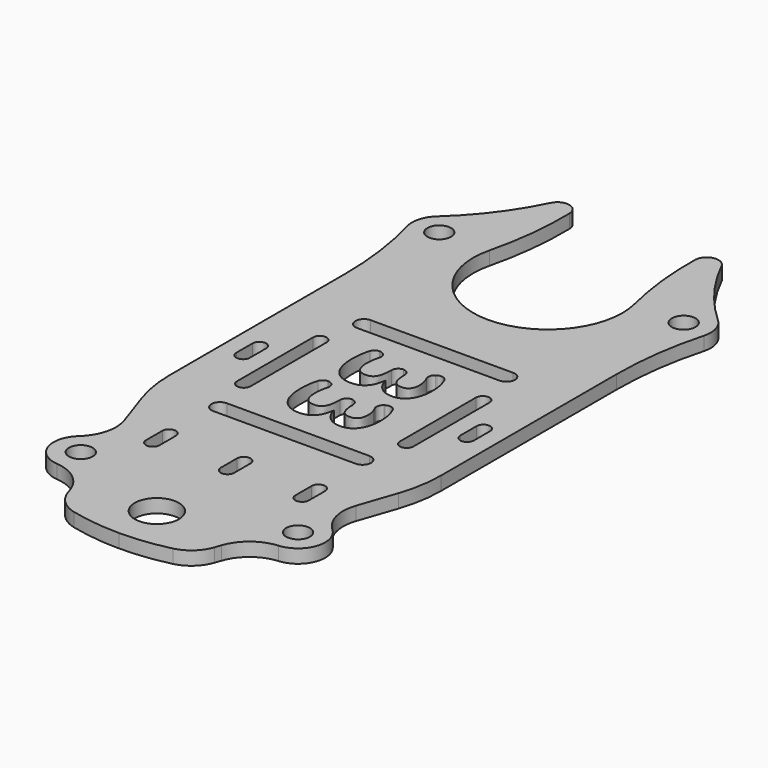
from build123d import *

# Parameters (mm, degrees)
F0_R        = 1.75
F0_R_2      = 3.25
F1_DEPTH    = 2
F2_T1_DEPTH = 2
F4_DEPTH    = 25


# Not quite as in the source:
# - a fillet or chamfer that OpenCascade refuses, or shapes differently, is made with other operations: its cross-section is extruded or revolved along the edge and cut away or added


with BuildPart() as f1:
    # F0 (on Top) → F1 (new body)
    with BuildSketch(Plane.XY):
        with BuildLine():
            ThreePointArc((-12.5713700234, 50.2695594093), (-16.118909248, 44.4802706126), (-20.6903729233, 39.460049583))
            ThreePointArc((-20.6903729233, 39.460049583), (-21.8414318775, 37.6150789796), (-21.8571428571, 35.4405430733))
            ThreePointArc((-21.8571428571, 35.4405430733), (-20.4663771338, 28.6163953155), (-20, 21.6676030258))
            Line((-20, 21.6676030258), (-20, -10.6856030045))
            ThreePointArc((-20, -10.6856030045), (-19.7308995433, -13.9554047127), (-18.9308396789, -17.1372159077))
            Line((-18.9308396789, -17.1372159077), (-17.0470641697, -22.6647409918))
            ThreePointArc((-17.0470641697, -22.6647409918), (-16.9162578432, -26.0979642803), (-18.6905264293, -29.0400899451))
            ThreePointArc((-18.6905264293, -29.0400899451), (-19.7861679358, -33.2903225806), (-16.3230484377, -35.9869336221))
            ThreePointArc((-16.3230484377, -35.9869336221), (-13.1213600073, -37.2332576723), (-11.1283691906, -40.0318501842))
            Line((-11.1283691906, -40.0318501842), (-10.837240035, -40.8861046865))
            ThreePointArc((-10.837240035, -40.8861046865), (-9.4747581102, -42.9666501557), (-7.2784782144, -44.1334325108))
            ThreePointArc((-7.2784782144, -44.1334325108), (-3.6649414842, -44.7825957956), (0, -45))
            ThreePointArc((0, -45), (3.6649414842, -44.7825957956), (7.2784782144, -44.1334325108))
            ThreePointArc((7.2784782144, -44.1334325108), (9.4747581102, -42.9666501557), (10.837240035, -40.8861046865))
            Line((10.837240035, -40.8861046865), (11.1283691906, -40.0318501842))
            ThreePointArc((11.1283691906, -40.0318501842), (13.1213600073, -37.2332576723), (16.3230484377, -35.9869336221))
            ThreePointArc((16.3230484377, -35.9869336221), (19.7861679358, -33.2903225806), (18.6905264293, -29.0400899451))
            ThreePointArc((18.6905264293, -29.0400899451), (16.9162578432, -26.0979642803), (17.0470641697, -22.6647409918))
            Line((17.0470641697, -22.6647409918), (18.9308396789, -17.1372159077))
            ThreePointArc((18.9308396789, -17.1372159077), (19.7308995433, -13.9554047127), (20, -10.6856030045))
            Line((20, -10.6856030045), (20, 21.6676030258))
            ThreePointArc((20, 21.6676030258), (20.4663771338, 28.6163953155), (21.8571428571, 35.4405430733))
            ThreePointArc((21.8571428571, 35.4405430733), (21.8414318775, 37.6150789796), (20.6903729233, 39.460049583))
            ThreePointArc((20.6903729233, 39.460049583), (16.118909248, 44.4802706126), (12.5713700234, 50.2695594093))
            ThreePointArc((12.5713700234, 50.2695594093), (10.6215560146, 51.2086657952), (9.25, 49.5345900586))
            ThreePointArc((9.25, 49.5345900586), (9.5452241746, 43.0321205381), (10.6826647736, 36.6231037599))
            ThreePointArc((10.6826647736, 36.6231037599), (8.6560424375, 27.2122957253), (0, 23))
            ThreePointArc((0, 23), (-8.6560424375, 27.2122957253), (-10.6826647736, 36.6231037599))
            ThreePointArc((-10.6826647736, 36.6231037599), (-9.5452241746, 43.0321205381), (-9.25, 49.5345900586))
            ThreePointArc((-9.25, 49.5345900586), (-10.6215560146, 51.2086657952), (-12.5713700234, 50.2695594093))
        make_face()
        with Locations((-16, -32)):
            Circle(F0_R, mode=Mode.SUBTRACT)
        with BuildLine():
            Line((-17.5, -1.5), (-17.5, 1.5))
            ThreePointArc((-17.5, 1.5), (-16.5, 2.5), (-15.5, 1.5))
            Line((-15.5, 1.5), (-15.5, -1.5))
            ThreePointArc((-15.5, -1.5), (-16.5, -2.5), (-17.5, -1.5))
        make_face(mode=Mode.SUBTRACT)
        with BuildLine():
            Line((-13, -7), (-13, 7))
            ThreePointArc((-13, 7), (-12, 8), (-11, 7))
            Line((-11, 7), (-11, -7))
            ThreePointArc((-11, -7), (-12, -8), (-13, -7))
        make_face(mode=Mode.SUBTRACT)
        with BuildLine():
            add(Edge.make_bspline(
                [(5.3190104167, -7.2317708333), (4.5703125, -8.3020833333), (3.2369791667, -8.3020833333)],
                knots=[0, 0, 0, 1, 1, 1], degree=2))
            add(Edge.make_bspline(
                [(3.2369791667, -8.3020833333), (2.1223958333, -8.3020833333), (1.3411458333, -7.6263020833)],
                knots=[0, 0, 0, 1, 1, 1], degree=2))
            add(Edge.make_bspline(
                [(1.3411458333, -7.6263020833), (0.5598958333, -6.9505208333), (0.265625, -5.7291666667)],
                knots=[0, 0, 0, 1, 1, 1], degree=2))
            Line((0.265625, -5.7291666667), (0.21875, -5.7291666667))
            add(Edge.make_bspline(
                [(0.21875, -5.7291666667), (0.0390625, -7.171875), (-0.6575520833, -7.9114583333)],
                knots=[0, 0, 0, 1, 1, 1], degree=2))
            add(Edge.make_bspline(
                [(-0.6575520833, -7.9114583333), (-1.3541666667, -8.6510416667), (-2.5338541667, -8.6510416667)],
                knots=[0, 0, 0, 1, 1, 1], degree=2))
            add(Edge.make_bspline(
                [(-2.5338541667, -8.6510416667), (-4.25, -8.6510416667), (-5.20703125, -7.40625)],
                knots=[0, 0, 0, 1, 1, 1], degree=2))
            add(Edge.make_bspline(
                [(-5.20703125, -7.40625), (-6.1640625, -6.1614583333), (-6.1640625, -3.8515625)],
                knots=[0, 0, 0, 1, 1, 1], degree=2))
            add(Edge.make_bspline(
                [(-6.1640625, -3.8515625), (-6.1640625, -1.9140625), (-5.5208333333, -0.4166666667)],
                knots=[0, 0, 0, 1, 1, 1], degree=2))
            Line((-5.5208333333, -0.4166666667), (-3.3802083333, -0.4166666667))
            add(Edge.make_bspline(
                [(-3.3802083333, -0.4166666667), (-3.7291666667, -1.1067708333), (-3.94921875, -1.9375)],
                knots=[0, 0, 0, 1, 1, 1], degree=2))
            add(Edge.make_bspline(
                [(-3.94921875, -1.9375), (-4.1692708333, -2.7682291667), (-4.1692708333, -3.5807291667)],
                knots=[0, 0, 0, 1, 1, 1], degree=2))
            add(Edge.make_bspline(
                [(-4.1692708333, -3.5807291667), (-4.1692708333, -4.828125), (-3.74609375, -5.421875)],
                knots=[0, 0, 0, 1, 1, 1], degree=2))
            add(Edge.make_bspline(
                [(-3.74609375, -5.421875), (-3.3229166667, -6.015625), (-2.3854166667, -6.015625)],
                knots=[0, 0, 0, 1, 1, 1], degree=2))
            add(Edge.make_bspline(
                [(-2.3854166667, -6.015625), (-1.5494791667, -6.015625), (-1.19921875, -5.33203125)],
                knots=[0, 0, 0, 1, 1, 1], degree=2))
            add(Edge.make_bspline(
                [(-1.19921875, -5.33203125), (-0.8489583333, -4.6484375), (-0.8489583333, -3.1510416667)],
                knots=[0, 0, 0, 1, 1, 1], degree=2))
            Line((-0.8489583333, -3.1510416667), (-0.8489583333, -2.2473958333))
            Line((-0.8489583333, -2.2473958333), (1.0807291667, -2.2473958333))
            Line((1.0807291667, -2.2473958333), (1.0807291667, -3.1666666667))
            add(Edge.make_bspline(
                [(1.0807291667, -3.1666666667), (1.0807291667, -4.5494791667), (1.4427083333, -5.1888020833)],
                knots=[0, 0, 0, 1, 1, 1], degree=2))
            add(Edge.make_bspline(
                [(1.4427083333, -5.1888020833), (1.8046875, -5.828125), (2.6822916667, -5.828125)],
                knots=[0, 0, 0, 1, 1, 1], degree=2))
            add(Edge.make_bspline(
                [(2.6822916667, -5.828125), (4.0338541667, -5.828125), (4.0338541667, -4.1354166667)],
                knots=[0, 0, 0, 1, 1, 1], degree=2))
            add(Edge.make_bspline(
                [(4.0338541667, -4.1354166667), (4.0338541667, -3.5494791667), (3.8385416667, -2.9427083333)],
                knots=[0, 0, 0, 1, 1, 1], degree=2))
            add(Edge.make_bspline(
                [(3.8385416667, -2.9427083333), (3.6432291667, -2.3359375), (3.1640625, -1.5963541667)],
                knots=[0, 0, 0, 1, 1, 1], degree=2))
            Line((3.1640625, -1.5963541667), (4.8958333333, -0.4322916667))
            add(Edge.make_bspline(
                [(4.8958333333, -0.4322916667), (6.0677083333, -2.0598958333), (6.0677083333, -4.3151041667)],
                knots=[0, 0, 0, 1, 1, 1], degree=2))
            add(Edge.make_bspline(
                [(6.0677083333, -4.3151041667), (6.0677083333, -6.1614583333), (5.3190104167, -7.2317708333)],
                knots=[0, 0, 0, 1, 1, 1], degree=2))
        make_face(mode=Mode.SUBTRACT)
        with Locations((0, -38)):
            Circle(F0_R_2, mode=Mode.SUBTRACT)
        with Locations((16, -32)):
            Circle(F0_R, mode=Mode.SUBTRACT)
        with BuildLine():
            Line((10.5, -14.5), (-10.5, -14.5))
            ThreePointArc((-10.5, -14.5), (-11.75, -13.25), (-10.5, -12))
            Line((-10.5, -12), (10.5, -12))
            ThreePointArc((10.5, -12), (11.75, -13.25), (10.5, -14.5))
        make_face(mode=Mode.SUBTRACT)
        with BuildLine():
            Line((11, -7), (11, 7))
            ThreePointArc((11, 7), (12, 8), (13, 7))
            Line((13, 7), (13, -7))
            ThreePointArc((13, -7), (12, -8), (11, -7))
        make_face(mode=Mode.SUBTRACT)
        with BuildLine():
            Line((15.5, -1.5), (15.5, 1.5))
            ThreePointArc((15.5, 1.5), (16.5, 2.5), (17.5, 1.5))
            Line((17.5, 1.5), (17.5, -1.5))
            ThreePointArc((17.5, -1.5), (16.5, -2.5), (15.5, -1.5))
        make_face(mode=Mode.SUBTRACT)
        with BuildLine():
            add(Edge.make_bspline(
                [(5.3190104167, 2.28125), (4.5703125, 1.2109375), (3.2369791667, 1.2109375)],
                knots=[0, 0, 0, 1, 1, 1], degree=2))
            add(Edge.make_bspline(
                [(3.2369791667, 1.2109375), (2.1223958333, 1.2109375), (1.3411458333, 1.88671875)],
                knots=[0, 0, 0, 1, 1, 1], degree=2))
            add(Edge.make_bspline(
                [(1.3411458333, 1.88671875), (0.5598958333, 2.5625), (0.265625, 3.7838541667)],
                knots=[0, 0, 0, 1, 1, 1], degree=2))
            Line((0.265625, 3.7838541667), (0.21875, 3.7838541667))
            add(Edge.make_bspline(
                [(0.21875, 3.7838541667), (0.0390625, 2.3411458333), (-0.6575520833, 1.6015625)],
                knots=[0, 0, 0, 1, 1, 1], degree=2))
            add(Edge.make_bspline(
                [(-0.6575520833, 1.6015625), (-1.3541666667, 0.8619791667), (-2.5338541667, 0.8619791667)],
                knots=[0, 0, 0, 1, 1, 1], degree=2))
            add(Edge.make_bspline(
                [(-2.5338541667, 0.8619791667), (-4.25, 0.8619791667), (-5.20703125, 2.1067708333)],
                knots=[0, 0, 0, 1, 1, 1], degree=2))
            add(Edge.make_bspline(
                [(-5.20703125, 2.1067708333), (-6.1640625, 3.3515625), (-6.1640625, 5.6614583333)],
                knots=[0, 0, 0, 1, 1, 1], degree=2))
            add(Edge.make_bspline(
                [(-6.1640625, 5.6614583333), (-6.1640625, 7.5989583333), (-5.5208333333, 9.0963541667)],
                knots=[0, 0, 0, 1, 1, 1], degree=2))
            Line((-5.5208333333, 9.0963541667), (-3.3802083333, 9.0963541667))
            add(Edge.make_bspline(
                [(-3.3802083333, 9.0963541667), (-3.7291666667, 8.40625), (-3.94921875, 7.5755208333)],
                knots=[0, 0, 0, 1, 1, 1], degree=2))
            add(Edge.make_bspline(
                [(-3.94921875, 7.5755208333), (-4.1692708333, 6.7447916667), (-4.1692708333, 5.9322916667)],
                knots=[0, 0, 0, 1, 1, 1], degree=2))
            add(Edge.make_bspline(
                [(-4.1692708333, 5.9322916667), (-4.1692708333, 4.6848958333), (-3.74609375, 4.0911458333)],
                knots=[0, 0, 0, 1, 1, 1], degree=2))
            add(Edge.make_bspline(
                [(-3.74609375, 4.0911458333), (-3.3229166667, 3.4973958333), (-2.3854166667, 3.4973958333)],
                knots=[0, 0, 0, 1, 1, 1], degree=2))
            add(Edge.make_bspline(
                [(-2.3854166667, 3.4973958333), (-1.5494791667, 3.4973958333), (-1.19921875, 4.1809895833)],
                knots=[0, 0, 0, 1, 1, 1], degree=2))
            add(Edge.make_bspline(
                [(-1.19921875, 4.1809895833), (-0.8489583333, 4.8645833333), (-0.8489583333, 6.3619791667)],
                knots=[0, 0, 0, 1, 1, 1], degree=2))
            Line((-0.8489583333, 6.3619791667), (-0.8489583333, 7.265625))
            Line((-0.8489583333, 7.265625), (1.0807291667, 7.265625))
            Line((1.0807291667, 7.265625), (1.0807291667, 6.3463541667))
            add(Edge.make_bspline(
                [(1.0807291667, 6.3463541667), (1.0807291667, 4.9635416667), (1.4427083333, 4.32421875)],
                knots=[0, 0, 0, 1, 1, 1], degree=2))
            add(Edge.make_bspline(
                [(1.4427083333, 4.32421875), (1.8046875, 3.6848958333), (2.6822916667, 3.6848958333)],
                knots=[0, 0, 0, 1, 1, 1], degree=2))
            add(Edge.make_bspline(
                [(2.6822916667, 3.6848958333), (4.0338541667, 3.6848958333), (4.0338541667, 5.3776041667)],
                knots=[0, 0, 0, 1, 1, 1], degree=2))
            add(Edge.make_bspline(
                [(4.0338541667, 5.3776041667), (4.0338541667, 5.9635416667), (3.8385416667, 6.5703125)],
                knots=[0, 0, 0, 1, 1, 1], degree=2))
            add(Edge.make_bspline(
                [(3.8385416667, 6.5703125), (3.6432291667, 7.1770833333), (3.1640625, 7.9166666667)],
                knots=[0, 0, 0, 1, 1, 1], degree=2))
            Line((3.1640625, 7.9166666667), (4.8958333333, 9.0807291667))
            add(Edge.make_bspline(
                [(4.8958333333, 9.0807291667), (6.0677083333, 7.453125), (6.0677083333, 5.1979166667)],
                knots=[0, 0, 0, 1, 1, 1], degree=2))
            add(Edge.make_bspline(
                [(6.0677083333, 5.1979166667), (6.0677083333, 3.3515625), (5.3190104167, 2.28125)],
                knots=[0, 0, 0, 1, 1, 1], degree=2))
        make_face(mode=Mode.SUBTRACT)
        with Locations((-18, 36.5)):
            Circle(F0_R, mode=Mode.SUBTRACT)
        with BuildLine():
            Line((10.5, 12), (-10.5, 12))
            ThreePointArc((-10.5, 12), (-11.75, 13.25), (-10.5, 14.5))
            Line((-10.5, 14.5), (10.5, 14.5))
            ThreePointArc((10.5, 14.5), (11.75, 13.25), (10.5, 12))
        make_face(mode=Mode.SUBTRACT)
        with Locations((18, 36.5)):
            Circle(F0_R, mode=Mode.SUBTRACT)
    extrude(amount=F1_DEPTH)

    # F2: fillet of radius 1 on 12 edges, made by hand

    # F2_s2 → F2_t1 (join)
    with BuildSketch(Plane.XY):
        with BuildLine():
            ThreePointArc((5.4823401509, 8.0731777614), (4.843595419, 8.6204570948), (4.0129893365, 8.4877806577))
            Line((4.0129893365, 8.4877806577), (3.9571236712, 8.5708917705))
            ThreePointArc((3.9571236712, 8.5708917705), (4.3986572425, 8.8672000385), (4.839967668, 9.1638402795))
            Line((4.839967668, 9.1638402795), (4.9771020437, 9.1392426381))
            ThreePointArc((4.9771020437, 9.1392426381), (5.3001177746, 8.6415597398), (5.573409567, 8.1148285845))
            Line((5.573409567, 8.1148285845), (5.4823401509, 8.0731777614))
        make_face()
        with BuildLine():
            ThreePointArc((3.9353958823, 8.4356238546), (3.5267558643, 7.8636788331), (3.5947276057, 7.1640449185))
            Line((3.5947276057, 7.1640449185), (3.5047965874, 7.119995944))
            ThreePointArc((3.5047965874, 7.119995944), (3.3039302948, 7.4968765259), (3.0800202169, 7.8622167368))
            Line((3.0800202169, 7.8622167368), (3.1081983093, 7.9997755857))
            ThreePointArc((3.1081983093, 7.9997755857), (3.4939765733, 8.2590881932), (3.8795316916, 8.5187327736))
            Line((3.8795316916, 8.5187327736), (3.9353958823, 8.4356238546))
        make_face()
        with BuildLine():
            ThreePointArc((1.0813955663, 6.2718756487), (0.7855723775, 6.9752785605), (0.0800558835, 7.266025))
            Line((0.0800558835, 7.266025), (0.0800558835, 7.3661615685))
            ThreePointArc((0.0800558835, 7.3661615685), (0.5803925251, 7.3657615685), (1.0807291667, 7.3657615685))
            Line((1.0807291667, 7.3657615685), (1.1808657352, 7.265625))
            ThreePointArc((1.1808657352, 7.265625), (1.1808657352, 6.3463541667), (1.1815295346, 6.2725972821))
            Line((1.1815295346, 6.2725972821), (1.0813955663, 6.2718756487))
        make_face()
        with BuildLine():
            ThreePointArc((0.1516589864, 7.266025), (-0.5538546526, 6.9752813949), (-0.8496806385, 6.2718836946))
            Line((-0.8496806385, 6.2718836946), (-0.9498146009, 6.2726061326))
            ThreePointArc((-0.9498146009, 6.2726061326), (-0.9490949019, 6.3619791667), (-0.9490949019, 7.265625))
            Line((-0.9490949019, 7.265625), (-0.8489583333, 7.3657615685))
            ThreePointArc((-0.8489583333, 7.3657615685), (-0.3486496735, 7.3657615685), (0.1516589864, 7.3661615685))
            Line((0.1516589864, 7.3661615685), (0.1516589864, 7.266025))
        make_face()
        with BuildLine():
            ThreePointArc((-3.8823882856, 7.8130958508), (-4.0409586866, 8.6953409018), (-4.8424375028, 9.0967541667))
            Line((-4.8424375028, 9.0967541667), (-4.8424375028, 9.1968381664))
            ThreePointArc((-4.8424375028, 9.1968381664), (-4.1113229181, 9.1964381664), (-3.3802083333, 9.1964381664))
            Line((-3.3802083333, 9.1964381664), (-3.2908936182, 9.0511912541))
            ThreePointArc((-3.2908936182, 9.0511912541), (-3.5673911757, 8.4298441391), (-3.7863833638, 7.784814019))
            Line((-3.7863833638, 7.784814019), (-3.8823882856, 7.8130958508))
        make_face()
        with BuildLine():
            ThreePointArc((-4.8235215119, 9.0967541667), (-5.4178362512, 8.9015689774), (-5.7807035945, 8.3920254967))
            Line((-5.7807035945, 8.3920254967), (-5.8764218027, 8.4217926297))
            ThreePointArc((-5.8764218027, 8.4217926297), (-5.7538395512, 8.7821164437), (-5.6129352586, 9.1359179502))
            Line((-5.6129352586, 9.1359179502), (-5.5208333333, 9.1965941667))
            ThreePointArc((-5.5208333333, 9.1965941667), (-5.1721774226, 9.1965941667), (-4.8235215119, 9.1969941667))
            Line((-4.8235215119, 9.1969941667), (-4.8235215119, 9.0967541667))
        make_face()
        with BuildLine():
            ThreePointArc((-3.8823882856, -1.6999249825), (-4.0409586866, -0.8176799315), (-4.8424375028, -0.4162666667))
            Line((-4.8424375028, -0.4162666667), (-4.8424375028, -0.3161826669))
            ThreePointArc((-4.8424375028, -0.3161826669), (-4.1113229181, -0.3165826669), (-3.3802083333, -0.3165826669))
            Line((-3.3802083333, -0.3165826669), (-3.2908936182, -0.4618295792))
            ThreePointArc((-3.2908936182, -0.4618295792), (-3.5673911757, -1.0831766942), (-3.7863833638, -1.7282068143))
            Line((-3.7863833638, -1.7282068143), (-3.8823882856, -1.6999249825))
        make_face()
        with BuildLine():
            ThreePointArc((-4.8235215119, -0.4162666667), (-5.4178362512, -0.611451856), (-5.7807035945, -1.1209953366))
            Line((-5.7807035945, -1.1209953366), (-5.8764218027, -1.0912282036))
            ThreePointArc((-5.8764218027, -1.0912282036), (-5.7538395512, -0.7309043896), (-5.6129352586, -0.3771028831))
            Line((-5.6129352586, -0.3771028831), (-5.5208333333, -0.3164266667))
            ThreePointArc((-5.5208333333, -0.3164266667), (-5.1721774226, -0.3164266667), (-4.8235215119, -0.3160266667))
            Line((-4.8235215119, -0.3160266667), (-4.8235215119, -0.4162666667))
        make_face()
        with BuildLine():
            ThreePointArc((0.1516589864, -2.2469958333), (-0.5538546526, -2.5377394384), (-0.8496806385, -3.2411371388))
            Line((-0.8496806385, -3.2411371388), (-0.9498146009, -3.2404147008))
            ThreePointArc((-0.9498146009, -3.2404147008), (-0.9490949019, -3.1510416667), (-0.9490949019, -2.2473958333))
            Line((-0.9490949019, -2.2473958333), (-0.8489583333, -2.1472592648))
            ThreePointArc((-0.8489583333, -2.1472592648), (-0.3486496735, -2.1472592648), (0.1516589864, -2.1468592648))
            Line((0.1516589864, -2.1468592648), (0.1516589864, -2.2469958333))
        make_face()
        with BuildLine():
            ThreePointArc((1.0813955663, -3.2411451846), (0.7855723775, -2.5377422728), (0.0800558835, -2.2469958333))
            Line((0.0800558835, -2.2469958333), (0.0800558835, -2.1468592648))
            ThreePointArc((0.0800558835, -2.1468592648), (0.5803925251, -2.1472592648), (1.0807291667, -2.1472592648))
            Line((1.0807291667, -2.1472592648), (1.1808657352, -2.2473958333))
            ThreePointArc((1.1808657352, -2.2473958333), (1.1808657352, -3.1666666667), (1.1815295346, -3.2404235512))
            Line((1.1815295346, -3.2404235512), (1.0813955663, -3.2411451846))
        make_face()
        with BuildLine():
            ThreePointArc((3.9353958823, -1.0773969787), (3.5267558643, -1.6493420003), (3.5947276057, -2.3489759148))
            Line((3.5947276057, -2.3489759148), (3.5047965874, -2.3930248894))
            ThreePointArc((3.5047965874, -2.3930248894), (3.3039302948, -2.0161443075), (3.0800202169, -1.6508040966))
            Line((3.0800202169, -1.6508040966), (3.1081983093, -1.5132452476))
            ThreePointArc((3.1081983093, -1.5132452476), (3.4939765733, -1.2539326401), (3.8795316916, -0.9942880597))
            Line((3.8795316916, -0.9942880597), (3.9353958823, -1.0773969787))
        make_face()
        with BuildLine():
            ThreePointArc((4.0129893365, -1.0252401757), (4.843595419, -0.8925637385), (5.4823401509, -1.439843072))
            Line((5.4823401509, -1.439843072), (5.573409567, -1.3981922488))
            ThreePointArc((5.573409567, -1.3981922488), (5.3001177746, -0.8714610935), (4.9771020437, -0.3737781952))
            Line((4.9771020437, -0.3737781952), (4.839967668, -0.3491805539))
            ThreePointArc((4.839967668, -0.3491805539), (4.3986572425, -0.6458207948), (3.9571236712, -0.9421290629))
            Line((3.9571236712, -0.9421290629), (4.0129893365, -1.0252401757))
        make_face()
    extrude(amount=F2_T1_DEPTH)

    # F3 (on face) → F4 (cut)
    with BuildSketch(Plane.XY.offset(2)):
        with BuildLine():
            ThreePointArc((12, -22), (11, -21), (10, -22))
            Line((10, -22), (10, -25))
            ThreePointArc((10, -25), (11, -26), (12, -25))
            Line((12, -25), (12, -22))
        make_face()
        with BuildLine():
            ThreePointArc((1, -22), (0, -21), (-1, -22))
            Line((-1, -22), (-1, -25))
            ThreePointArc((-1, -25), (0, -26), (1, -25))
            Line((1, -25), (1, -22))
        make_face()
        with BuildLine():
            Line((-10, -25), (-10, -22))
            ThreePointArc((-10, -22), (-11, -21), (-12, -22))
            Line((-12, -22), (-12, -25))
            ThreePointArc((-12, -25), (-11, -26), (-10, -25))
        make_face()
    extrude(amount=-F4_DEPTH, mode=Mode.SUBTRACT)


solid = f1.part
